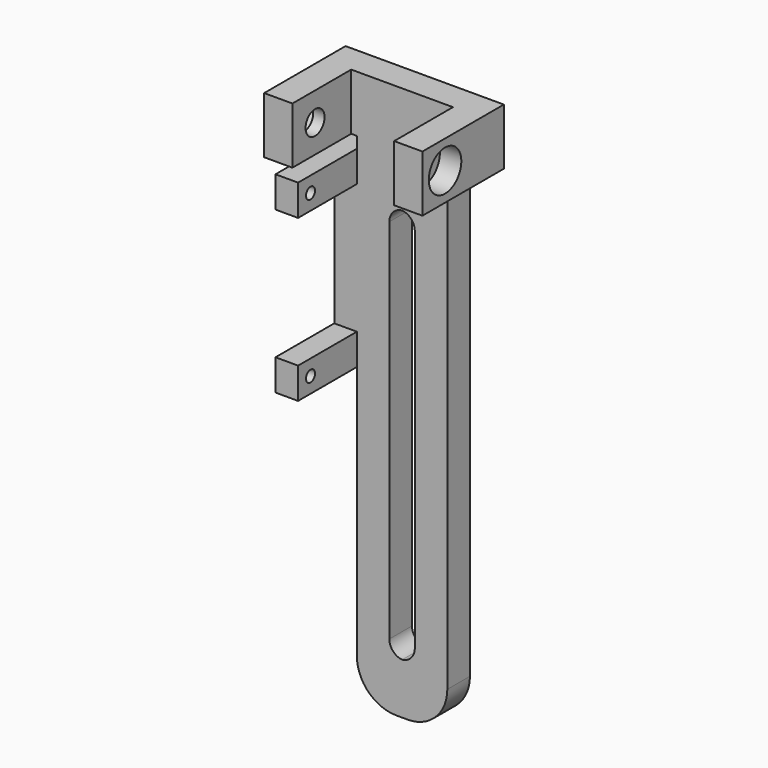
from build123d import *

# Parameters (mm, degrees)
F0_W         = 4.5
F0_H         = 70
F0_W_2       = 4
F0_H_2       = 34
F1_DEPTH     = 5
F2_W         = 5
F2_H         = 10
F2_W_2       = 4
F2_H_2       = 5.5
F3_DEPTH     = 13
F4_R         = 2.1
F4_R_2       = 1
F5_DEPTH     = 28.001
F6_R         = 2.1
F7_DEPTH     = 3
F8_R         = 3.6
F8_R_2       = 2.1
F9_DEPTH     = 3.8
F10_R        = 7
F11_T1_DEPTH = 5


# Not quite as in the source:
# - a fillet or chamfer that OpenCascade refuses, or shapes differently, is made with other operations: its cross-section is extruded or revolved along the edge and cut away or added


with BuildPart() as f1:
    # F0 (on Front) → F1 (new body)
    with BuildSketch(Plane.XZ):
        Polygon((-8, -44), (8, -44), (8, 44), (-8, 44), (-8, 42), (-8, 8), align=None)
        Rectangle(F0_W, F0_H, mode=Mode.SUBTRACT)
        Polygon((-8, 44), (8, 44), (14, 44), (14, 54), (-14, 54), (-14, 44), align=None)
        with Locations((-10, 25)):
            Rectangle(F0_W_2, F0_H_2)
    extrude(amount=F1_DEPTH)

    # F2 (on face) → F3 (join)
    with BuildSketch(Plane.XZ.offset(5)):
        with Locations((11.5, 49)):
            Rectangle(F2_W, F2_H)
        with Locations((-11.5, 49)):
            Rectangle(F2_W, F2_H)
        with Locations((-10, 10.75)):
            Rectangle(F2_W_2, F2_H_2)
        with Locations((-10, 39.25)):
            Rectangle(F2_W_2, F2_H_2)
    extrude(amount=F3_DEPTH)

    # F4 (on face) → F5 (cut, through all)
    with BuildSketch(Plane(origin=(-14, 0, 0), x_dir=(0, -1, 0), z_dir=(-1, 0, 0))):
        with Locations((13, 49)):
            Circle(F4_R)
        with Locations((15.25, 39.25)):
            Circle(F4_R_2)
        with Locations((15.25, 10.75)):
            Circle(F4_R_2)
    extrude(amount=-F5_DEPTH, mode=Mode.SUBTRACT)

    # F6 (on face) → F7 (cut)
    with BuildSketch(Plane(origin=(-14, 0, 0), x_dir=(0, -1, 0), z_dir=(-1, 0, 0))):
        Polygon((15.0784609691, 45.4), (17.1569219382, 49), (15.0784609691, 52.6), (10.9215390309, 52.6), (8.8430780618, 49), (10.9215390309, 45.4), align=None)
        with Locations((13, 49)):
            Circle(F6_R, mode=Mode.SUBTRACT)
    extrude(amount=-F7_DEPTH, mode=Mode.SUBTRACT)

    # F8 (on face) → F9 (cut)
    with BuildSketch(Plane.YZ.offset(14)):
        with Locations((-13, 49)):
            Circle(F8_R)
        with Locations((-13, 49)):
            Circle(F8_R_2, mode=Mode.SUBTRACT)
    extrude(amount=-F9_DEPTH, mode=Mode.SUBTRACT)

    # F10
    f10_edges = [f1.edges().sort_by_distance(p)[0] for p in [
        (8, -2.5, -44),
        (-8, -2.5, -44),
    ]]
    fillet(f10_edges, radius=F10_R)

    # F11: fillet of radius 2.5 on 4 edges, made by hand

    # F11_s2 → F11_t1 (join)
    with BuildSketch(Plane.XZ):
        with BuildLine():
            ThreePointArc((0.25, -35), (-1.517766953, -34.267766953), (-2.25, -32.5))
            Line((-2.25, -32.5), (-2.25, -35))
            Line((-2.25, -35), (0.25, -35))
        make_face()
        with BuildLine():
            ThreePointArc((2.25, -32.5), (1.517766953, -34.267766953), (-0.25, -35))
            Line((-0.25, -35), (2.25, -35))
            Line((2.25, -35), (2.25, -32.5))
        make_face()
        with BuildLine():
            ThreePointArc((-2.25, 32.5), (-1.517766953, 34.267766953), (0.25, 35))
            Line((0.25, 35), (-2.25, 35))
            Line((-2.25, 35), (-2.25, 32.5))
        make_face()
        with BuildLine():
            ThreePointArc((2.25, 32.5), (1.517766953, 34.267766953), (-0.25, 35))
            Line((-0.25, 35), (2.25, 35))
            Line((2.25, 35), (2.25, 32.5))
        make_face()
    extrude(amount=F11_T1_DEPTH)


solid = f1.part
